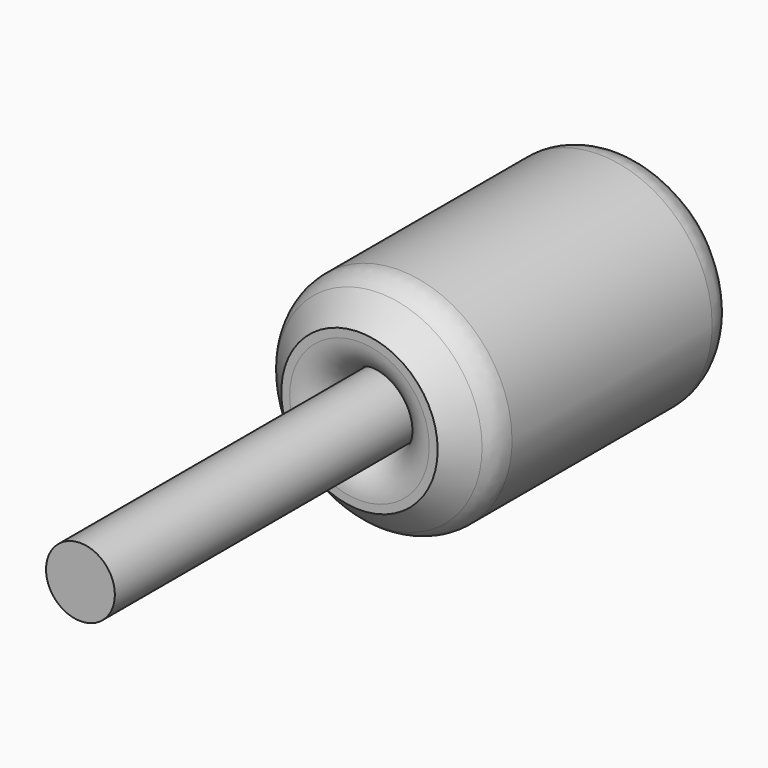
from build123d import *

# Parameters (mm, degrees)
F0_R     = 3.2421303212
F1_DEPTH = 10
F2_SIZE  = 1
F4_D     = 2
F5_R     = 1
F6_R     = 0.9870539352
F7_DEPTH = 20


with BuildPart() as f1:
    # F0 (on Front) → F1 (new body)
    with BuildSketch(Plane.XZ):
        Circle(F0_R)
    extrude(amount=F1_DEPTH)

    # F2
    f2_edges = [f1.edges().sort_by_distance(p)[0] for p in [
        (3.24213, -5, 0),
        (-3.24213, 0, 0),
        (-3.24213, -10, 0),
    ]]
    chamfer(f2_edges, length=F2_SIZE)

    # F4 (through all)
    with Locations(Plane(origin=(0, 0, 0), x_dir=(1, 0, 0), z_dir=(0, 1, 0))):
        with Locations((0, 0)):
            Hole(F4_D / 2)

    # F5
    f5_edges = [f1.edges().sort_by_distance(p)[0] for p in [
        (-3.24213, -9, 0),
        (-3.24213, -1, 0),
        (2.74213, -0.5, 0),
        (-2.24213, 0, 0),
        (-1, -10, 0),
    ]]
    fillet(f5_edges, radius=F5_R)


with BuildPart() as f7:
    # F6 (on Front) → F7 (new body)
    with BuildSketch(Plane.XZ):
        Circle(F6_R)
    extrude(amount=F7_DEPTH)


solid = Compound([f1.part, f7.part])
